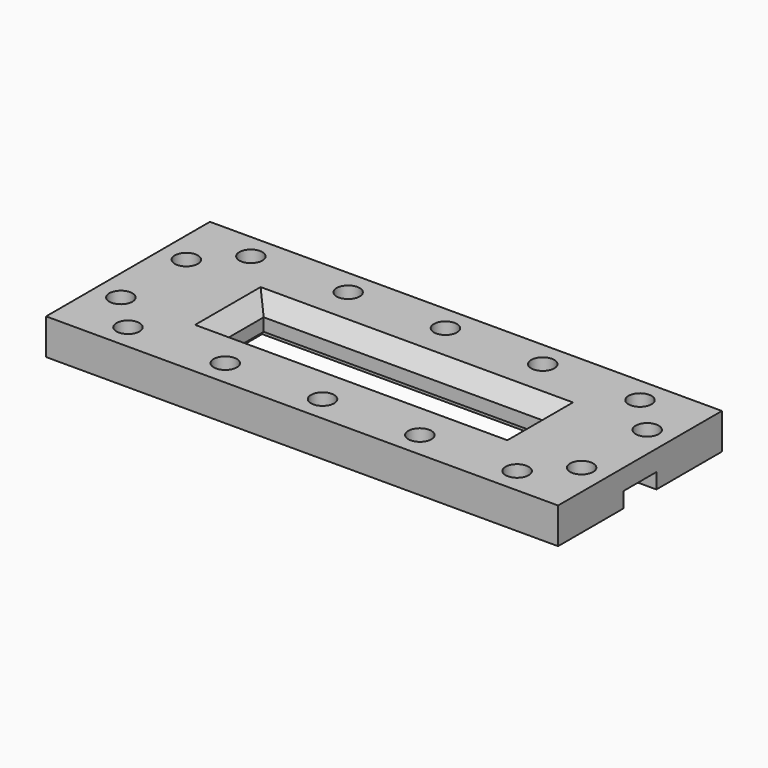
from build123d import *

# Parameters (mm, degrees)
F0_W      = 100
F0_H      = 40
F1_DEPTH  = 7
F2_W      = 55
F2_H      = 10
F3_DEPTH  = 8
F4_SIZE   = 3
F5_R      = 2.25
F6_DEPTH  = 18.9
F7_W      = 18
F7_H      = 8
F8_DEPTH  = 3
F9_W      = 55
F9_H      = 10
F10_DEPTH = 1.5
F12_DEPTH = 0.5


# Not quite as in the source:
# - a feature names something its author has since deleted; it is built from what else it names


with BuildPart() as f1:
    # F0 (on Top) → F1 (new body)
    with BuildSketch(Plane.XY):
        with Locations((50, -20)):
            Rectangle(F0_W, F0_H)
    extrude(amount=F1_DEPTH)

    # F2 (on Top) → F3 (cut)
    with BuildSketch(Plane.XY):
        with Locations((50, -20)):
            Rectangle(F2_W, F2_H)
    extrude(amount=F3_DEPTH, mode=Mode.SUBTRACT)

    # F4
    f4_edges = [f1.edges().sort_by_distance(p)[0] for p in [
        (50, -15, 7),
        (22.5, -20, 7),
        (50, -25, 7),
        (77.5, -20, 7),
    ]]
    chamfer(f4_edges, length=F4_SIZE)

    # F5 (on Top) → F6 (cut)
    with BuildSketch(Plane.XY):
        with Locations((12, -35)):
            Circle(F5_R)
        with Locations((31, -35)):
            Circle(F5_R)
        with Locations((50, -35)):
            Circle(F5_R)
        with Locations((69, -35)):
            Circle(F5_R)
        with Locations((88, -35)):
            Circle(F5_R)
        with Locations((95, -28)):
            Circle(F5_R)
        with Locations((95, -12)):
            Circle(F5_R)
        with Locations((88, -5)):
            Circle(F5_R)
        with Locations((69, -5)):
            Circle(F5_R)
        with Locations((50, -5)):
            Circle(F5_R)
        with Locations((31, -5)):
            Circle(F5_R)
        with Locations((12, -5)):
            Circle(F5_R)
        with Locations((5, -12)):
            Circle(F5_R)
        with Locations((5, -28)):
            Circle(F5_R)
    extrude(amount=F6_DEPTH, mode=Mode.SUBTRACT)

    # F7 (on face) → F8 (cut)
    with BuildSketch(Plane(origin=(0, 0, 0), x_dir=(1, 0, 0), z_dir=(0, 0, -1))):
        with Locations((9, 20)):
            Rectangle(F7_W, F7_H)
        with Locations((91, 20)):
            Rectangle(F7_W, F7_H)
    extrude(amount=-F8_DEPTH, mode=Mode.SUBTRACT)

    # F9 (on face) → F10 (cut)
    with BuildSketch(Plane(origin=(0, 0, 0), x_dir=(1, 0, 0), z_dir=(0, 0, -1))):
        Polygon((21, 13.5), (77.5, 13.5), (79, 13.5), (79, 26.5), (21, 26.5), align=None)
        with Locations((50, 20)):
            Rectangle(F9_W, F9_H, mode=Mode.SUBTRACT)
    extrude(amount=-F10_DEPTH, mode=Mode.SUBTRACT)

    # F11 (on face) → F12 (cut)
    with BuildSketch(Plane(origin=(0, 0, 0), x_dir=(1, 0, 0), z_dir=(0, 0, -1))):
        with BuildLine():
            Line((14, 8.5), (16, 8.5))
            Line((16, 8.5), (84, 8.5))
            Line((84, 8.5), (86, 8.5))
            ThreePointArc((86, 8.5), (88.1213203436, 9.3786796564), (89, 11.5))
            Line((89, 11.5), (89, 16))
            Line((89, 16), (87, 16))
            Line((87, 16), (87, 11.5))
            ThreePointArc((87, 11.5), (86.7071067812, 10.7928932188), (86, 10.5))
            Line((86, 10.5), (84, 10.5))
            Line((84, 10.5), (16, 10.5))
            Line((16, 10.5), (14, 10.5))
            ThreePointArc((14, 10.5), (13.2928932188, 10.7928932188), (13, 11.5))
            Line((13, 11.5), (13, 16))
            Line((13, 16), (11, 16))
            Line((11, 16), (11, 11.5))
            ThreePointArc((11, 11.5), (11.8786796564, 9.3786796564), (14, 8.5))
        make_face()
        with BuildLine():
            Line((11, 28.5), (11, 24))
            Line((11, 24), (13, 24))
            Line((13, 24), (13, 28.5))
            ThreePointArc((13, 28.5), (13.2928932188, 29.2071067812), (14, 29.5))
            Line((14, 29.5), (16, 29.5))
            Line((16, 29.5), (84, 29.5))
            Line((84, 29.5), (86, 29.5))
            ThreePointArc((86, 29.5), (86.7071067812, 29.2071067812), (87, 28.5))
            Line((87, 28.5), (87, 24))
            Line((87, 24), (89, 24))
            Line((89, 24), (89, 28.5))
            ThreePointArc((89, 28.5), (88.1213203436, 30.6213203436), (86, 31.5))
            Line((86, 31.5), (84, 31.5))
            Line((84, 31.5), (16, 31.5))
            Line((16, 31.5), (14, 31.5))
            ThreePointArc((14, 31.5), (11.8786796564, 30.6213203436), (11, 28.5))
        make_face()
    extrude(amount=-F12_DEPTH, mode=Mode.SUBTRACT)


solid = f1.part
